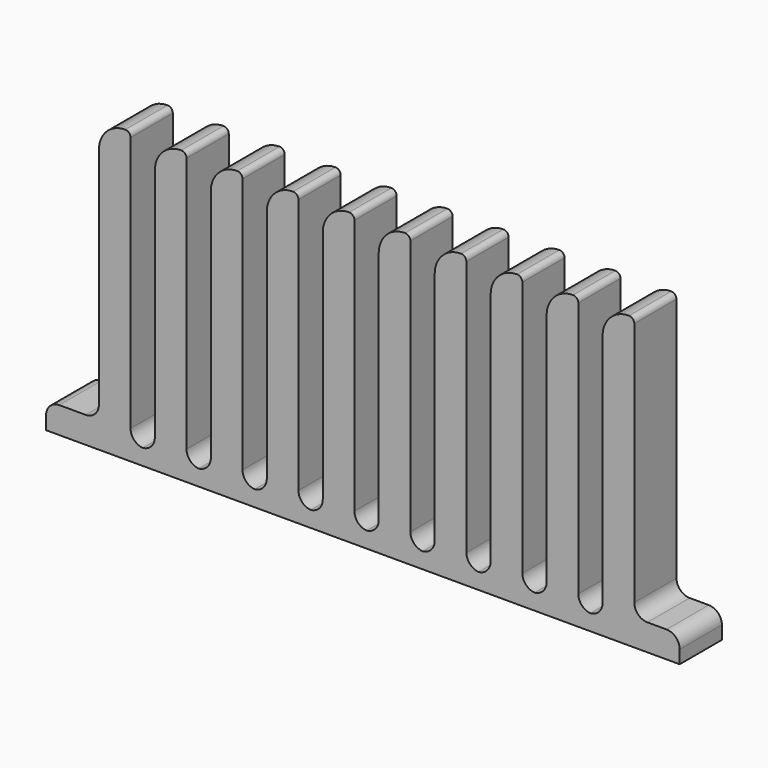
from build123d import *

# Parameters (mm, degrees)
F0_W        = 120
F0_H        = 10
F1_DEPTH    = 5
F2_W        = 6
F2_H        = 10
F3_DEPTH    = 50
F4_W        = 4.6
F4_H        = 10
F5_DEPTH    = 2
F6_T1_DEPTH = 10
F6_T3_DEPTH = 22.5
F7_R        = 5
F8_R        = 0.99999


# Not quite as in the source:
# - a fillet or chamfer that OpenCascade refuses, or shapes differently, is made with other operations: its cross-section is extruded or revolved along the edge and cut away or added
# - a fillet or chamfer is up to 0.001 mm smaller than in the source, because OpenCascade refuses the exact size


with BuildPart() as f1:
    # F0 (on Top) → F1 (new body)
    with BuildSketch(Plane.XY):
        with Locations((-1.1, -55)):
            Rectangle(F0_W, F0_H)
    extrude(amount=F1_DEPTH)

    # F2 (on face) → F3 (join)
    with BuildSketch(Plane.XY.offset(5)):
        with Locations((-48.1, -55)):
            Rectangle(F2_W, F2_H)
        with Locations((-37.5, -55)):
            Rectangle(F2_W, F2_H)
        with Locations((-26.9, -55)):
            Rectangle(F2_W, F2_H)
        with Locations((-16.3, -55)):
            Rectangle(F2_W, F2_H)
        with Locations((-5.7, -55)):
            Rectangle(F2_W, F2_H)
        with Locations((4.9, -55)):
            Rectangle(F2_W, F2_H)
        with Locations((15.5, -55)):
            Rectangle(F2_W, F2_H)
        with Locations((26.1, -55)):
            Rectangle(F2_W, F2_H)
        with Locations((36.7, -55)):
            Rectangle(F2_W, F2_H)
        with Locations((47.3, -55)):
            Rectangle(F2_W, F2_H)
    extrude(amount=F3_DEPTH)

    # F4 (on face) → F5 (cut)
    with BuildSketch(Plane.XY.offset(5)):
        with Locations((-42.8, -55)):
            Rectangle(F4_W, F4_H)
        with Locations((-32.2, -55)):
            Rectangle(F4_W, F4_H)
        with Locations((-21.6, -55)):
            Rectangle(F4_W, F4_H)
        with Locations((-11, -55)):
            Rectangle(F4_W, F4_H)
        with Locations((-0.4, -55)):
            Rectangle(F4_W, F4_H)
        with Locations((10.2, -55)):
            Rectangle(F4_W, F4_H)
        with Locations((20.8, -55)):
            Rectangle(F4_W, F4_H)
        with Locations((31.4, -55)):
            Rectangle(F4_W, F4_H)
        with Locations((42, -55)):
            Rectangle(F4_W, F4_H)
    extrude(amount=-F5_DEPTH, mode=Mode.SUBTRACT)

    # F6: fillet of radius 2.5 on 22 edges, made by hand

    # F6_s2 → F6_t1 (join)
    with BuildSketch(Plane.XZ.offset(50)):
        with BuildLine():
            ThreePointArc((-45.1, 5.5), (-44.367766953, 3.732233047), (-42.6, 3))
            Line((-42.6, 3), (-45.1, 3))
            Line((-45.1, 3), (-45.1, 5.5))
        make_face()
        with BuildLine():
            ThreePointArc((-43, 3), (-41.232233047, 3.732233047), (-40.5, 5.5))
            Line((-40.5, 5.5), (-40.5, 3))
            Line((-40.5, 3), (-43, 3))
        make_face()
        with BuildLine():
            ThreePointArc((-32.4, 3), (-30.632233047, 3.732233047), (-29.9, 5.5))
            Line((-29.9, 5.5), (-29.9, 3))
            Line((-29.9, 3), (-32.4, 3))
        make_face()
        with BuildLine():
            ThreePointArc((-23.9, 5.5), (-23.167766953, 3.732233047), (-21.4, 3))
            Line((-21.4, 3), (-23.9, 3))
            Line((-23.9, 3), (-23.9, 5.5))
        make_face()
        with BuildLine():
            ThreePointArc((-21.8, 3), (-20.032233047, 3.732233047), (-19.3, 5.5))
            Line((-19.3, 5.5), (-19.3, 3))
            Line((-19.3, 3), (-21.8, 3))
        make_face()
        with BuildLine():
            ThreePointArc((-13.3, 5.5), (-12.567766953, 3.732233047), (-10.8, 3))
            Line((-10.8, 3), (-13.3, 3))
            Line((-13.3, 3), (-13.3, 5.5))
        make_face()
        with BuildLine():
            ThreePointArc((-11.2, 3), (-9.432233047, 3.732233047), (-8.7, 5.5))
            Line((-8.7, 5.5), (-8.7, 3))
            Line((-8.7, 3), (-11.2, 3))
        make_face()
        with BuildLine():
            ThreePointArc((-2.7, 5.5), (-1.967766953, 3.732233047), (-0.2, 3))
            Line((-0.2, 3), (-2.7, 3))
            Line((-2.7, 3), (-2.7, 5.5))
        make_face()
        with BuildLine():
            ThreePointArc((-0.6, 3), (1.167766953, 3.732233047), (1.9, 5.5))
            Line((1.9, 5.5), (1.9, 3))
            Line((1.9, 3), (-0.6, 3))
        make_face()
        with BuildLine():
            ThreePointArc((10, 3), (11.767766953, 3.732233047), (12.5, 5.5))
            Line((12.5, 5.5), (12.5, 3))
            Line((12.5, 3), (10, 3))
        make_face()
        with BuildLine():
            ThreePointArc((20.6, 3), (22.367766953, 3.732233047), (23.1, 5.5))
            Line((23.1, 5.5), (23.1, 3))
            Line((23.1, 3), (20.6, 3))
        make_face()
        with BuildLine():
            ThreePointArc((31.2, 3), (32.967766953, 3.732233047), (33.7, 5.5))
            Line((33.7, 5.5), (33.7, 3))
            Line((33.7, 3), (31.2, 3))
        make_face()
        with BuildLine():
            ThreePointArc((41.8, 3), (43.567766953, 3.732233047), (44.3, 5.5))
            Line((44.3, 5.5), (44.3, 3))
            Line((44.3, 3), (41.8, 3))
        make_face()
        with BuildLine():
            ThreePointArc((39.7, 5.5), (40.432233047, 3.732233047), (42.2, 3))
            Line((42.2, 3), (39.7, 3))
            Line((39.7, 3), (39.7, 5.5))
        make_face()
        with BuildLine():
            ThreePointArc((29.1, 5.5), (29.832233047, 3.732233047), (31.6, 3))
            Line((31.6, 3), (29.1, 3))
            Line((29.1, 3), (29.1, 5.5))
        make_face()
        with BuildLine():
            ThreePointArc((18.5, 5.5), (19.232233047, 3.732233047), (21, 3))
            Line((21, 3), (18.5, 3))
            Line((18.5, 3), (18.5, 5.5))
        make_face()
        with BuildLine():
            ThreePointArc((7.9, 5.5), (8.632233047, 3.732233047), (10.4, 3))
            Line((10.4, 3), (7.9, 3))
            Line((7.9, 3), (7.9, 5.5))
        make_face()
        with BuildLine():
            ThreePointArc((50.3, 7.5), (51.032233047, 5.732233047), (52.8, 5))
            Line((52.8, 5), (50.3, 5))
            Line((50.3, 5), (50.3, 7.5))
        make_face()
        with BuildLine():
            ThreePointArc((-53.6, 5), (-51.832233047, 5.732233047), (-51.1, 7.5))
            Line((-51.1, 7.5), (-51.1, 5))
            Line((-51.1, 5), (-53.6, 5))
        make_face()
        with BuildLine():
            ThreePointArc((-34.5, 5.5), (-33.767766953, 3.732233047), (-32, 3))
            Line((-32, 3), (-34.5, 3))
            Line((-34.5, 3), (-34.5, 5.5))
        make_face()
    extrude(amount=F6_T1_DEPTH)

    # F6_s4 → F6_t3 (cut)
    with BuildSketch(Plane.XZ.offset(43.75)):
        with BuildLine():
            ThreePointArc((58.9, 2.5), (58.167766953, 4.267766953), (56.4, 5))
            Line((56.4, 5), (58.9, 5))
            Line((58.9, 5), (58.9, 2.5))
        make_face()
        with BuildLine():
            ThreePointArc((-58.6, 5), (-60.367766953, 4.267766953), (-61.1, 2.5))
            Line((-61.1, 2.5), (-61.1, 5))
            Line((-61.1, 5), (-58.6, 5))
        make_face()
    extrude(amount=F6_T3_DEPTH, mode=Mode.SUBTRACT)

    # F7
    f7_edges = [f1.edges().sort_by_distance(p)[0] for p in [
        (-51.1, -55, 55),
        (-40.5, -55, 55),
        (-29.9, -55, 55),
        (-19.3, -55, 55),
        (-8.7, -55, 55),
        (1.9, -55, 55),
        (12.5, -55, 55),
        (23.1, -55, 55),
        (33.7, -55, 55),
        (44.3, -55, 55),
    ]]
    fillet(f7_edges, radius=F7_R)

    # F8 (radius 1 in the source; OpenCascade refuses exactly that, so slightly less here)
    f8_edges = [f1.edges().sort_by_distance(p)[0] for p in [
        (-45.1, -55, 55),
        (-34.5, -55, 55),
        (-23.9, -55, 55),
        (-13.3, -55, 55),
        (-2.7, -55, 55),
        (7.9, -55, 55),
        (18.5, -55, 55),
        (29.1, -55, 55),
        (39.7, -55, 55),
        (50.3, -55, 55),
    ]]
    fillet(f8_edges, radius=F8_R)


solid = f1.part
